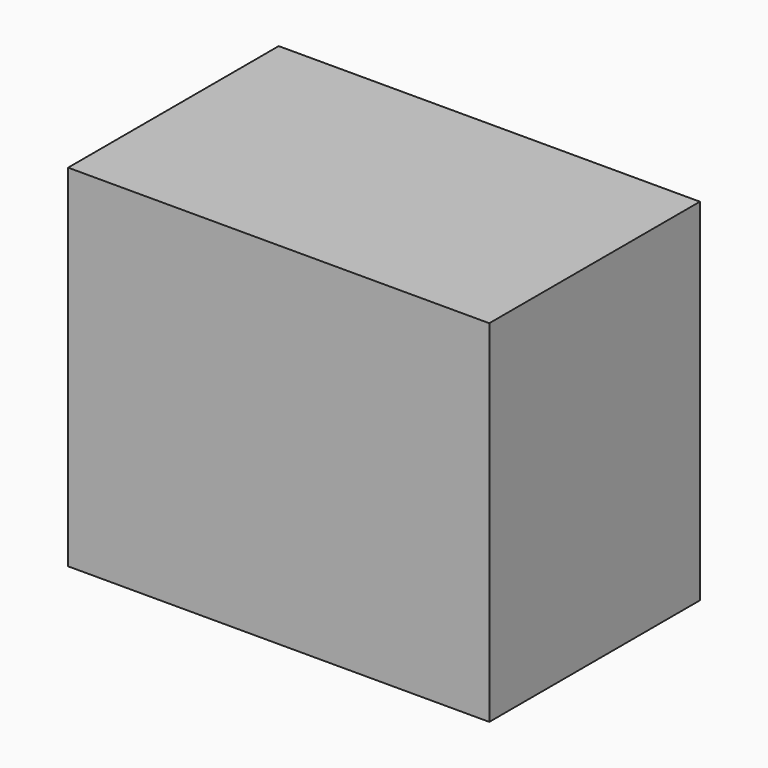
from build123d import *

# Parameters (mm, degrees)
F0_W     = 19.05
F0_H     = 1.27
F3_DEPTH = 15.24
F4_ANGLE = 90


# Not quite as in the source:
# - a feature names something its author has since deleted; it is built from what else it names
# - the program builds the solid bodies; features that only make, move or delete a surface that nothing else refers to are left out


with BuildPart() as f3:
    # F0 (on Front) → F3 (new body, symmetric)
    with BuildSketch(Plane.XZ):
        with Locations((0, 12.065)):
            Rectangle(F0_W, F0_H)
        with Locations((0, 10.795)):
            Rectangle(F0_W, F0_H)
        with Locations((0, 9.525)):
            Rectangle(F0_W, F0_H)
        with Locations((0, 8.255)):
            Rectangle(F0_W, F0_H)
        with Locations((0, 6.985)):
            Rectangle(F0_W, F0_H)
        with Locations((0, 5.715)):
            Rectangle(F0_W, F0_H)
        with Locations((0, 4.445)):
            Rectangle(F0_W, F0_H)
        with Locations((0, 3.175)):
            Rectangle(F0_W, F0_H)
        with Locations((0, 1.905)):
            Rectangle(F0_W, F0_H)
        with Locations((0, 0.635)):
            Rectangle(F0_W, F0_H)
        with Locations((0, -0.635)):
            Rectangle(F0_W, F0_H)
        with Locations((0, -1.905)):
            Rectangle(F0_W, F0_H)
        with Locations((0, -3.175)):
            Rectangle(F0_W, F0_H)
        with Locations((0, -4.445)):
            Rectangle(F0_W, F0_H)
        with Locations((0, -5.715)):
            Rectangle(F0_W, F0_H)
        with Locations((0, -6.985)):
            Rectangle(F0_W, F0_H)
        with Locations((0, -8.255)):
            Rectangle(F0_W, F0_H)
        with Locations((0, -9.525)):
            Rectangle(F0_W, F0_H)
        with Locations((0, -10.795)):
            Rectangle(F0_W, F0_H)
        with Locations((0, -12.065)):
            Rectangle(F0_W, F0_H)
    extrude(amount=F3_DEPTH, both=True)


with BuildPart() as f3_1:
    # F4: moved
    add(f3.part.rotate(Axis((9.525, 15.24, 0), (0, 0, 1)), F4_ANGLE))


solid = f3_1.part
